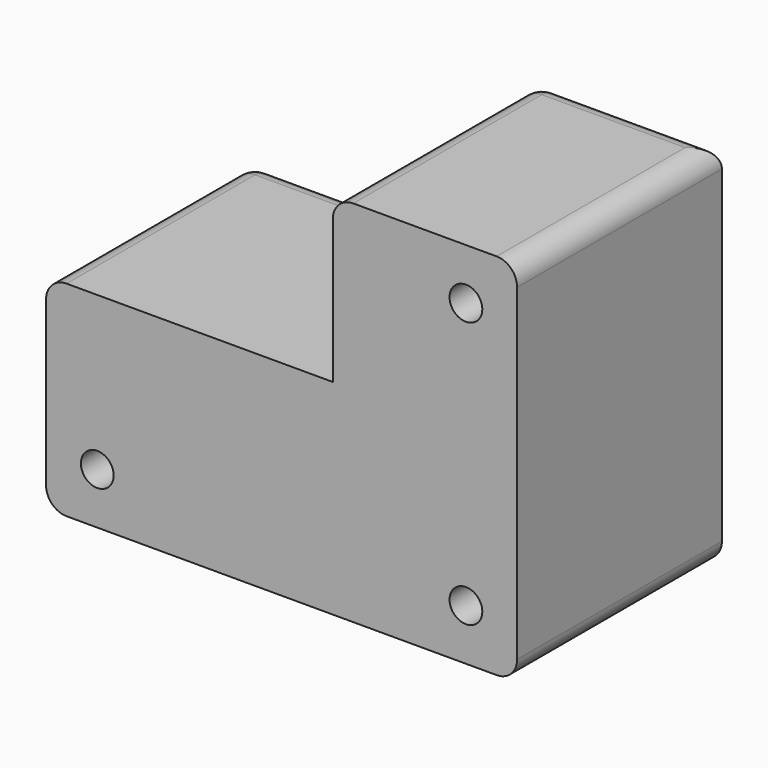
from build123d import *

# Parameters (mm, degrees)
F0_R         = 3.25
F0_R_2       = 1.6
F0_W         = 26
F0_H         = 2
F1_DEPTH     = 25
F2_DEPTH     = 15
F3_T1_DEPTH  = 23
F3_T3_DEPTH  = 21
F3_T5_DEPTH  = 28
F3_T7_DEPTH  = 35
F3_T9_DEPTH  = 26
F3_T11_DEPTH = 14
F3_S15_W     = 2
F3_S15_H     = 2
F3_T16_DEPTH = 2
F3_S21_W     = 2
F3_S21_H     = 2
F3_T22_DEPTH = 2
F3_T29_DEPTH = 31
F3_T33_DEPTH = 19


# Not quite as in the source:
# - a fillet or chamfer that OpenCascade refuses, or shapes differently, is made with other operations: its cross-section is extruded or revolved along the edge and cut away or added


with BuildPart() as f1:
    # F0 (on Front) → F1 (new body)
    with BuildSketch(Plane.XZ):
        Polygon((-23, 0), (-23, -18), (23, -18), (23, 18), (5, 18), (5, 2), (3, 2), (3, 0), align=None)
        with Locations((-18, -13)):
            Circle(F0_R, mode=Mode.SUBTRACT)
        with Locations((18, -13)):
            Circle(F0_R, mode=Mode.SUBTRACT)
        with Locations((18, 13)):
            Circle(F0_R, mode=Mode.SUBTRACT)
        with Locations((18, 13)):
            Circle(F0_R)
        with Locations((18, 13)):
            Circle(F0_R_2, mode=Mode.SUBTRACT)
        with Locations((18, -13)):
            Circle(F0_R)
        with Locations((18, -13)):
            Circle(F0_R_2, mode=Mode.SUBTRACT)
        with Locations((-18, -13)):
            Circle(F0_R)
        with Locations((-18, -13)):
            Circle(F0_R_2, mode=Mode.SUBTRACT)
        with Locations((-10, 1)):
            Rectangle(F0_W, F0_H)
    extrude(amount=F1_DEPTH)

    # F0 (on Front) → F2 (cut)
    with BuildSketch(Plane.XZ):
        with Locations((18, -13)):
            Circle(F0_R)
        with Locations((18, -13)):
            Circle(F0_R_2, mode=Mode.SUBTRACT)
        with Locations((-18, -13)):
            Circle(F0_R)
        with Locations((-18, -13)):
            Circle(F0_R_2, mode=Mode.SUBTRACT)
        with Locations((18, 13)):
            Circle(F0_R)
        with Locations((18, 13)):
            Circle(F0_R_2, mode=Mode.SUBTRACT)
    extrude(amount=F2_DEPTH, mode=Mode.SUBTRACT)

    # F3: fillet of radius 2 on 9 edges, made by hand

    # F3_s2 → F3_t1 (cut)
    with BuildSketch(Plane.XY.offset(-23)):
        with BuildLine():
            ThreePointArc((-23, -2), (-22.4142135624, -0.5857864376), (-21, 0))
            Line((-21, 0), (-23, 0))
            Line((-23, 0), (-23, -2))
        make_face()
    extrude(amount=F3_T1_DEPTH, mode=Mode.SUBTRACT)

    # F3_s4 → F3_t3 (cut)
    with BuildSketch(Plane.YZ.offset(7)):
        with BuildLine():
            ThreePointArc((0, 16), (-0.5857864376, 17.4142135624), (-2, 18))
            Line((-2, 18), (0, 18))
            Line((0, 18), (0, 16))
        make_face()
    extrude(amount=F3_T3_DEPTH, mode=Mode.SUBTRACT)

    # F3_s6 → F3_t5 (cut)
    with BuildSketch(Plane.XZ.offset(2)):
        with BuildLine():
            ThreePointArc((-23, 0), (-22.4142135624, 1.4142135624), (-21, 2))
            Line((-21, 2), (-23, 2))
            Line((-23, 2), (-23, 0))
        make_face()
        with BuildLine():
            ThreePointArc((7, 18), (5.5857864376, 17.4142135624), (5, 16))
            Line((5, 16), (5, 18))
            Line((5, 18), (7, 18))
        make_face()
    extrude(amount=F3_T5_DEPTH, mode=Mode.SUBTRACT)

    # F3_s8 → F3_t7 (cut)
    with BuildSketch(Plane.XZ.offset(-5)):
        with BuildLine():
            ThreePointArc((-21, -18), (-22.4142135624, -17.4142135624), (-23, -16))
            Line((-23, -16), (-23, -18))
            Line((-23, -18), (-21, -18))
        make_face()
        with BuildLine():
            ThreePointArc((21, -18), (22.4142135624, -17.4142135624), (23, -16))
            Line((23, -16), (23, -18))
            Line((23, -18), (21, -18))
        make_face()
        with BuildLine():
            ThreePointArc((23, 16), (22.4142135624, 17.4142135624), (21, 18))
            Line((21, 18), (23, 18))
            Line((23, 18), (23, 16))
        make_face()
    extrude(amount=F3_T7_DEPTH, mode=Mode.SUBTRACT)

    # F3_s10 → F3_t9 (cut)
    with BuildSketch(Plane.YZ.offset(-21)):
        with BuildLine():
            ThreePointArc((0, 0), (-0.5857864376, 1.4142135624), (-2, 2))
            Line((-2, 2), (0, 2))
            Line((0, 2), (0, 0))
        make_face()
    extrude(amount=F3_T9_DEPTH, mode=Mode.SUBTRACT)

    # F3_s12 → F3_t11 (cut)
    with BuildSketch(Plane.XY.offset(2)):
        with BuildLine():
            ThreePointArc((7, 0), (5.5857864376, -0.5857864376), (5, -2))
            Line((5, -2), (5, 0))
            Line((5, 0), (7, 0))
        make_face()
    extrude(amount=F3_T11_DEPTH, mode=Mode.SUBTRACT)


with BuildPart() as f3_tool14:
    # F3_s15 → F3_t16 (new body)
    with BuildSketch(Plane.YZ.offset(-21)):
        with Locations((-1, 1)):
            Rectangle(F3_S15_W, F3_S15_H)
    extrude(amount=-F3_T16_DEPTH)

    # F3_s17 → F3_t18 (revolve, cut)
    with BuildSketch(Plane(origin=(-21, -2, 0), x_dir=(0, -0.7071067812, -0.7071067812), z_dir=(0, 0.7071067812, -0.7071067812))):
        with BuildLine():
            ThreePointArc((0, -2), (2, 0), (0, 2))
            Line((0, 2), (0, -2))
        make_face()
    revolve(axis=Axis((-21, -2, 0), (-1, 0, 0)), mode=Mode.SUBTRACT)


with BuildPart() as f1_1:
    add(f1.part)

    # F3_t13: cut F3_tool14
    add(f3_tool14.part, mode=Mode.SUBTRACT)


with BuildPart() as f3_tool20:
    # F3_s21 → F3_t22 (new body)
    with BuildSketch(Plane.XZ.offset(2)):
        with Locations((6, 17)):
            Rectangle(F3_S21_W, F3_S21_H)
    extrude(amount=-F3_T22_DEPTH)

    # F3_s23 → F3_t24 (revolve, cut)
    with BuildSketch(Plane(origin=(7, -2, 16), x_dir=(0.7071067812, 0, -0.7071067812), z_dir=(0.7071067812, 0, 0.7071067812))):
        with BuildLine():
            ThreePointArc((0, -2), (2, 0), (0, 2))
            Line((0, 2), (0, -2))
        make_face()
    revolve(axis=Axis((7, -2, 16), (0, 1, 0)), mode=Mode.SUBTRACT)


with BuildPart() as f1_2:
    add(f1_1.part)

    # F3_t19: cut F3_tool20
    add(f3_tool20.part, mode=Mode.SUBTRACT)


with BuildPart() as f3_tool27:
    # F3_s28 → F3_t29 (new body)
    with BuildSketch(Plane.YZ.offset(10)):
        with BuildLine():
            ThreePointArc((0, 0), (-0.5857864376, 1.4142135624), (-2, 2))
            Line((-2, 2), (0, 2))
            Line((0, 2), (0, 0))
        make_face()
    extrude(amount=-F3_T29_DEPTH)

    split(bisect_by=Plane.YZ.offset(5), keep=Keep.TOP)


with BuildPart() as f3_tool31:
    # F3_s32 → F3_t33 (new body)
    with BuildSketch(Plane.XY.offset(16)):
        with BuildLine():
            ThreePointArc((7, 0), (5.5857864376, -0.5857864376), (5, -2))
            Line((5, -2), (5, 0))
            Line((5, 0), (7, 0))
        make_face()
    extrude(amount=-F3_T33_DEPTH)

    split(bisect_by=Plane.XY.offset(2), keep=Keep.BOTTOM)


with BuildPart() as f3_tool27_1:
    add(f3_tool27.part)

    # F3_t35: intersect F3_tool31
    add(f3_tool31.part, mode=Mode.INTERSECT)


with BuildPart() as f1_3:
    add(f1_2.part)

    # F3_t25: cut F3_tool27
    add(f3_tool27_1.part, mode=Mode.SUBTRACT)


solid = f1_3.part
